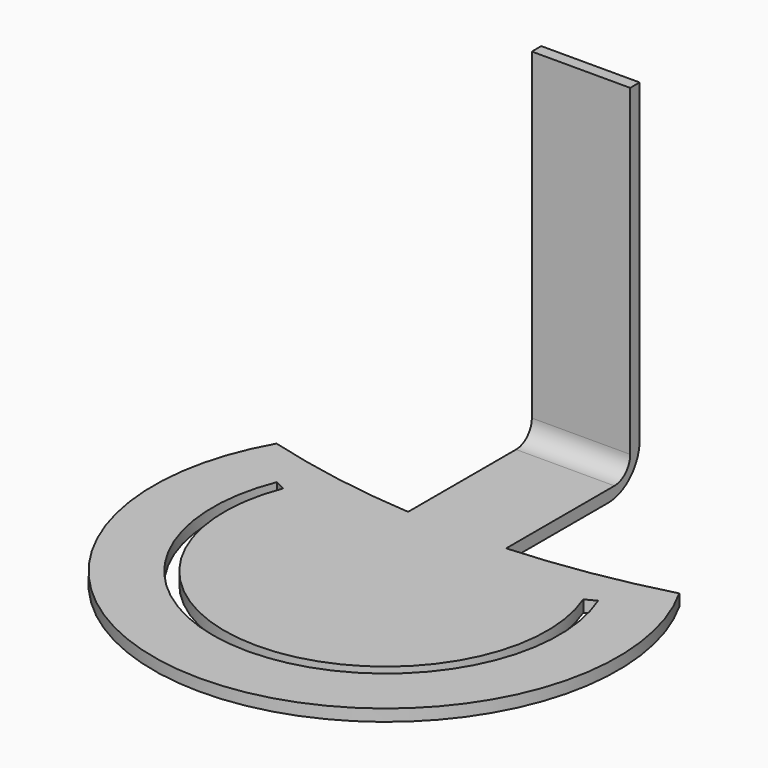
from build123d import *

# Parameters (mm, degrees)
F0_W     = 50
F0_H     = 6
F2_DEPTH = 130
F0_H_2   = 100
F0_H_3   = 74
F3_DEPTH = 6
F4_R     = 20
F5_R     = 10
F7_DEPTH = 6
F9_DEPTH = 31


# Not quite as in the source:
# - a feature names something its author has since deleted; it is built from what else it names


with BuildPart() as f2:
    # F0 (on Front) → F2 (new body)
    with BuildSketch(Plane.XZ):
        with Locations((-5, -147)):
            Rectangle(F0_W, F0_H)
    extrude(amount=F2_DEPTH)

    # F0 (on Front) → F3 (join)
    with BuildSketch(Plane.XZ):
        with Locations((-5, -20)):
            Rectangle(F0_W, F0_H_2)
        with Locations((-5, -107)):
            Rectangle(F0_W, F0_H_3)
        with Locations((-5, -147)):
            Rectangle(F0_W, F0_H)
    extrude(amount=F3_DEPTH)

    # F4
    f4_edges = [f2.edges().sort_by_distance(p)[0] for p in [
        (-5, 0, -150),
    ]]
    fillet(f4_edges, radius=F4_R)

    # F5
    f5_edges = [f2.edges().sort_by_distance(p)[0] for p in [
        (-5, -6, -144),
    ]]
    fillet(f5_edges, radius=F5_R)

    # F6 (on face) → F7 (join)
    with BuildSketch(Plane.XY.offset(-144)):
        with BuildLine():
            ThreePointArc((-30, -84.6159367699), (-69.042085877, -79.9604861418), (-107.415399673, -71.3903940482))
            ThreePointArc((-107.415399673, -71.3903940482), (-5.4112498239, -247.9992833605), (97.8214378821, -72.1056832508))
            ThreePointArc((97.8214378821, -72.1056832508), (59.233233327, -80.4336085853), (20, -84.8105109003))
            Line((20, -84.8105109003), (20, -130))
            Line((20, -130), (-30, -130))
            Line((-30, -130), (-30, -84.6159367699))
        make_face()
    extrude(amount=-F7_DEPTH)

    # F8 (on face) → F9 (cut)
    with BuildSketch(Plane.XY.offset(-144)):
        with BuildLine():
            Line((-81.2895118016, -99.9348974879), (-86.618032779, -97.1768430661))
            ThreePointArc((-86.618032779, -97.1768430661), (-77.8915033239, -179.2513111401), (-5, -217.9708071228))
            ThreePointArc((-5, -217.9708071228), (67.8915033239, -179.2513111401), (76.618032779, -97.1768430661))
            Line((76.618032779, -97.1768430661), (71.2895118016, -99.9348974879))
            ThreePointArc((71.2895118016, -99.9348974879), (62.7839892821, -176.1446724661), (-5, -212))
            ThreePointArc((-5, -212), (-72.7839892821, -176.1446724661), (-81.2895118016, -99.9348974879))
        make_face()
    extrude(amount=-F9_DEPTH, mode=Mode.SUBTRACT)


solid = f2.part
